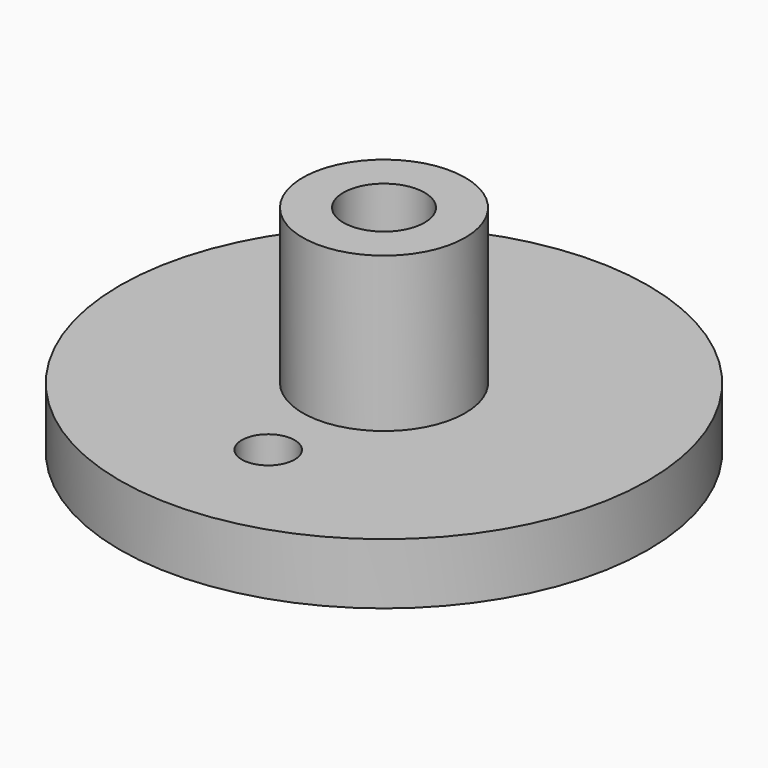
from build123d import *

# Parameters (mm, degrees)
F0_R     = 6.5
F0_R_2   = 1
F1_DEPTH = 1.5
F2_R     = 2
F2_R_2   = 1
F3_DEPTH = 3.8
F4_R     = 0.6498381819
F5_DEPTH = 1.5


# Not quite as in the source:
# - a feature names something its author has since deleted; it is built from what else it names


with BuildPart() as f1:
    # F0 (on Top) → F1 (new body)
    with BuildSketch(Plane.XY):
        Circle(F0_R)
        Circle(F0_R_2, mode=Mode.SUBTRACT)
    extrude(amount=F1_DEPTH)

    # F2 (on face) → F3 (join)
    with BuildSketch(Plane.XY.offset(1.5)):
        Circle(F2_R)
        Circle(F2_R_2, mode=Mode.SUBTRACT)
    extrude(amount=F3_DEPTH)

    # F4 (on Top) → F5 (cut, through all)
    with BuildSketch(Plane.XY):
        with Locations((0, -3.5616646055)):
            Circle(F4_R)
    extrude(amount=F5_DEPTH, mode=Mode.SUBTRACT)


solid = f1.part
